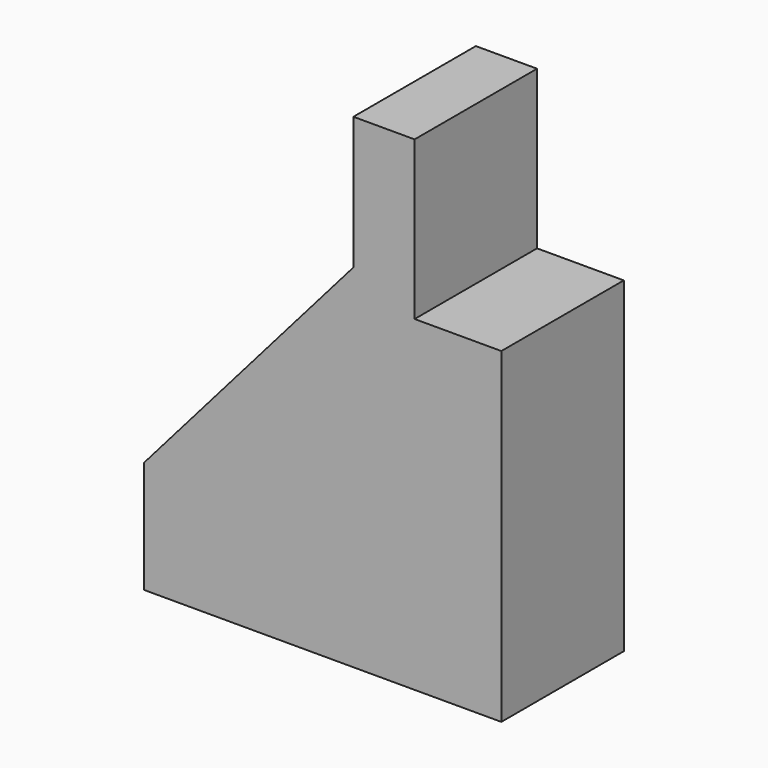
from build123d import *

# Parameters (mm, degrees)
F0_W      = 70
F0_H      = 30
F1_DEPTH  = 95
F2_W      = 17
F2_H      = 31
F3_DEPTH  = 41.4
F4_R      = 9.75
F5_DEPTH  = 60
F8_DEPTH  = 43.7
F6_R      = 7.5
F9_DEPTH  = 57
F10_R     = 9.75
F11_DEPTH = 40
F12_R     = 9.75
F13_DEPTH = 20
F14_R     = 7.5
F15_DEPTH = 32.1
F16_R     = 7.5
F17_DEPTH = 11.1
F19_DEPTH = 25


# Not quite as in the source:
# - a feature names something its author has since deleted; it is built from what else it names


with BuildPart() as f1:
    # F0 (on Top) → F1 (new body)
    with BuildSketch(Plane.XY):
        with Locations((22, 0)):
            Rectangle(F0_W, F0_H)
    extrude(amount=F1_DEPTH)

    # F2 (on face) → F3 (cut)
    with BuildSketch(Plane.XZ.offset(15)):
        with Locations((48.5, 79.5)):
            Rectangle(F2_W, F2_H)
    extrude(amount=-F3_DEPTH, mode=Mode.SUBTRACT)

    # F4 (on face) → F5 (cut)
    with BuildSketch(Plane(origin=(0, 0, 0), x_dir=(1, 0, 0), z_dir=(0, 0, -1))):
        with Locations((44, 0)):
            Circle(F4_R)
    extrude(amount=-F5_DEPTH, mode=Mode.SUBTRACT)

    # F7 (on face) → F8 (cut)
    with BuildSketch(Plane(origin=(0, 15, 0), x_dir=(-1, 0, 0), z_dir=(0, 1, 0))):
        Polygon((13, 95), (-28, 95), (-28, 69), (13, 22), align=None)
    extrude(amount=-F8_DEPTH, mode=Mode.SUBTRACT)

    # F6 (on face) → F9 (cut)
    with BuildSketch(Plane(origin=(-13, 0, 0), x_dir=(0, -1, 0), z_dir=(-1, 0, 0))):
        with Locations((0, 52)):
            Circle(F6_R)
    extrude(amount=-F9_DEPTH, mode=Mode.SUBTRACT)

    # F10 (on face) → F11 (cut)
    with BuildSketch(Plane(origin=(0, 0, 0), x_dir=(1, 0, 0), z_dir=(0, 0, -1))):
        with Locations((22, 0)):
            Circle(F10_R)
    extrude(amount=-F11_DEPTH, mode=Mode.SUBTRACT)

    # F12 (on face) → F13 (cut)
    with BuildSketch(Plane(origin=(0, 0, 0), x_dir=(1, 0, 0), z_dir=(0, 0, -1))):
        Circle(F12_R)
    extrude(amount=-F13_DEPTH, mode=Mode.SUBTRACT)

    # F14 (on face) → F15 (cut)
    with BuildSketch(Plane(origin=(-13, 0, 0), x_dir=(0, -1, 0), z_dir=(-1, 0, 0))):
        with Locations((0, 32)):
            Circle(F14_R)
    extrude(amount=-F15_DEPTH, mode=Mode.SUBTRACT)

    # F16 (on face) → F17 (cut)
    with BuildSketch(Plane(origin=(-13, 0, 0), x_dir=(0, -1, 0), z_dir=(-1, 0, 0))):
        with Locations((0, 12)):
            Circle(F16_R)
    extrude(amount=-F17_DEPTH, mode=Mode.SUBTRACT)

    # F18 (on face) → F19 (cut)
    with BuildSketch(Plane(origin=(-13, 0, 0), x_dir=(0, -1, 0), z_dir=(-1, 0, 0))):
        with BuildLine():
            Line((-7.5, 42), (-7.5, 32))
            ThreePointArc((-7.5, 32), (0, 24.5), (7.5, 32))
            Line((7.5, 32), (7.5, 42))
            Line((7.5, 42), (-7.5, 42))
        make_face()
    extrude(amount=-F19_DEPTH, mode=Mode.SUBTRACT)


solid = f1.part
